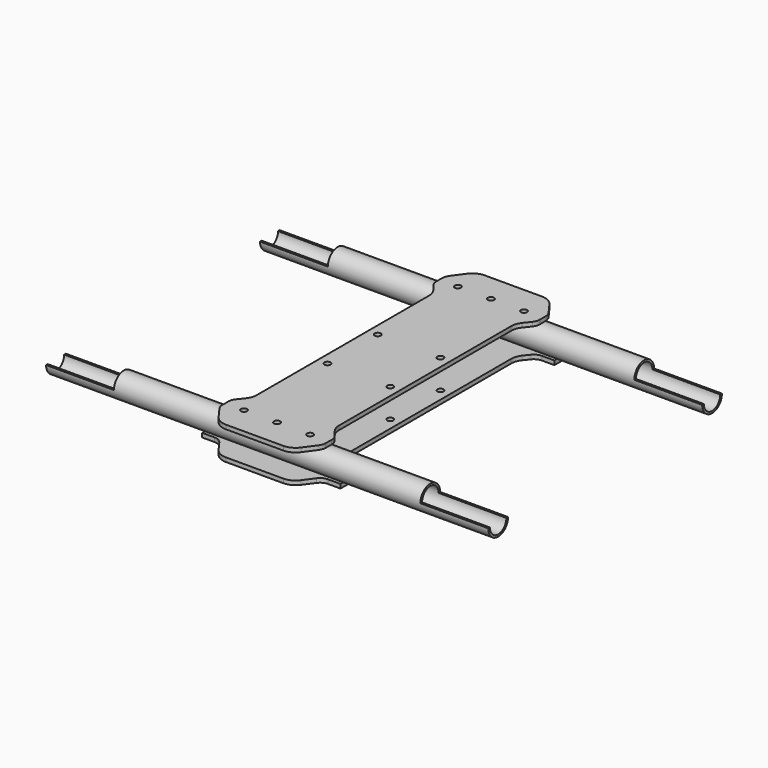
from build123d import *

# Parameters (mm, degrees)
F1_R     = 6
F1_R_2   = 5
F2_DEPTH = 107.5
F4_START = -6
F3_R     = 1.5
F4_DEPTH = 2
F6_START = 6
F5_R     = 1.5
F6_DEPTH = 2
F7_W     = 33
F7_H     = 12
F8_DEPTH = 6
F9_R     = 5
F9_2_R   = 5
F10_R    = 7.4575999994
F10_2_R  = 7.4575999994


with BuildPart() as f2:
    # F1 (on Right) → F2 (new body, symmetric)
    with BuildSketch(Plane.YZ):
        with Locations((-65, 0)):
            Circle(F1_R)
        with Locations((-65, 0)):
            Circle(F1_R_2, mode=Mode.SUBTRACT)
    extrude(amount=F2_DEPTH, both=True)


with BuildPart() as f2b:
    # F1 (on Right) → F2, piece 2 (new body, symmetric)
    with BuildSketch(Plane.YZ):
        with Locations((65, 0)):
            Circle(F1_R)
        with Locations((65, 0)):
            Circle(F1_R_2, mode=Mode.SUBTRACT)
    extrude(amount=F2_DEPTH, both=True)


with BuildPart() as f4:
    # F3 (on Top) → F4 (new body)
    with BuildSketch(Plane.XY.offset(F4_START)):
        Polygon((-20, 0), (-20, -54.9247604212), (-25.1882806771, -61.5001681654), (-33.6882806771, -61.5001681654), (-33.6196620251, -68.4998318346), (-25.1196620251, -68.4998318346), (-17.7541729063, -78.6235332489), (0, -78.6235332489), (17.7541729063, -78.6235332489), (25.1196620251, -68.4998318346), (33.6196620251, -68.4998318346), (33.6882806771, -61.5001681654), (25.1882806771, -61.5001681654), (20, -54.9247604212), (20, 0), (20, 54.9247604212), (25.1882806771, 61.5001681654), (33.6882806771, 61.5001681654), (33.6196620251, 68.4998318346), (25.1196620251, 68.4998318346), (17.7541729063, 78.6235332489), (0, 78.6235332489), (-17.7541729063, 78.6235332489), (-25.1196620251, 68.4998318346), (-33.6196620251, 68.4998318346), (-33.6882806771, 61.5001681654), (-25.1882806771, 61.5001681654), (-20, 54.9247604212), align=None)
        with Locations((-16.0910124415, -65)):
            Circle(F3_R, mode=Mode.SUBTRACT)
        with Locations((-15.25, -15.25)):
            Circle(F3_R, mode=Mode.SUBTRACT)
        with Locations((0, -65)):
            Circle(F3_R, mode=Mode.SUBTRACT)
        with Locations((16.0910124415, -65)):
            Circle(F3_R, mode=Mode.SUBTRACT)
        with Locations((15.25, -15.25)):
            Circle(F3_R, mode=Mode.SUBTRACT)
        with Locations((-15.25, 15.25)):
            Circle(F3_R, mode=Mode.SUBTRACT)
        with Locations((-16.0910124415, 65)):
            Circle(F3_R, mode=Mode.SUBTRACT)
        with Locations((15.25, 15.25)):
            Circle(F3_R, mode=Mode.SUBTRACT)
        with Locations((0, 65)):
            Circle(F3_R, mode=Mode.SUBTRACT)
        with Locations((16.0910124415, 65)):
            Circle(F3_R, mode=Mode.SUBTRACT)
    extrude(amount=-F4_DEPTH)

    # F9
    f9_edges = [f4.edges().sort_by_distance(p)[0] for p in [
        (-25.119662, -68.499832, -7),
        (25.119662, -68.499832, -7),
        (25.188281, -61.500168, -7),
        (-25.188281, -61.500168, -7),
        (-25.119662, 68.499832, -7),
        (25.119662, 68.499832, -7),
        (25.188281, 61.500168, -7),
        (-25.188281, 61.500168, -7),
    ]]
    fillet(f9_edges, radius=F9_R)

    # F10
    f10_edges = [f4.edges().sort_by_distance(p)[0] for p in [
        (17.754173, 78.623533, -7),
        (-17.754173, 78.623533, -7),
        (-20, 54.92476, -7),
        (20, 54.92476, -7),
        (20, -54.92476, -7),
        (17.754173, -78.623533, -7),
        (-17.754173, -78.623533, -7),
        (-20, -54.92476, -7),
    ]]
    fillet(f10_edges, radius=F10_R)


with BuildPart() as f6:
    # F5 (on Top) → F6 (new body)
    with BuildSketch(Plane.XY.offset(F6_START)):
        Polygon((-20, 0), (-20, -54.9247604212), (-25.1882806771, -61.5001681654), (-25.1196620251, -68.4998318346), (-17.7541729063, -78.6235332489), (0, -78.6235332489), (17.7541729063, -78.6235332489), (25.1196620251, -68.4998318346), (25.1882806771, -61.5001681654), (20, -54.9247604212), (20, 0), (20, 54.9247604212), (25.1882806771, 61.5001681654), (25.1196620251, 68.4998318346), (17.7541729063, 78.6235332489), (0, 78.6235332489), (-17.7541729063, 78.6235332489), (-25.1196620251, 68.4998318346), (-25.1882806771, 61.5001681654), (-20, 54.9247604212), align=None)
        with Locations((-16.0910124415, -65)):
            Circle(F5_R, mode=Mode.SUBTRACT)
        with Locations((-15.25, -15.25)):
            Circle(F5_R, mode=Mode.SUBTRACT)
        with Locations((0, -65)):
            Circle(F5_R, mode=Mode.SUBTRACT)
        with Locations((16.0910124415, -65)):
            Circle(F5_R, mode=Mode.SUBTRACT)
        with Locations((15.25, -15.25)):
            Circle(F5_R, mode=Mode.SUBTRACT)
        with Locations((-15.25, 15.25)):
            Circle(F5_R, mode=Mode.SUBTRACT)
        with Locations((-16.0910124415, 65)):
            Circle(F5_R, mode=Mode.SUBTRACT)
        with Locations((15.25, 15.25)):
            Circle(F5_R, mode=Mode.SUBTRACT)
        with Locations((0, 65)):
            Circle(F5_R, mode=Mode.SUBTRACT)
        with Locations((16.0910124415, 65)):
            Circle(F5_R, mode=Mode.SUBTRACT)
    extrude(amount=F6_DEPTH)

    # F9#2
    f9_2_edges = [f6.edges().sort_by_distance(p)[0] for p in [
        (-25.119662, 68.499832, 7),
        (-25.188281, 61.500168, 7),
        (25.119662, 68.499832, 7),
        (25.188281, 61.500168, 7),
        (25.119662, -68.499832, 7),
        (25.188281, -61.500168, 7),
        (-25.188281, -61.500168, 7),
        (-25.119662, -68.499832, 7),
    ]]
    fillet(f9_2_edges, radius=F9_2_R)

    # F10#2
    f10_2_edges = [f6.edges().sort_by_distance(p)[0] for p in [
        (-17.754173, 78.623533, 7),
        (17.754173, 78.623533, 7),
        (20, -54.92476, 7),
        (20, 54.92476, 7),
        (17.754173, -78.623533, 7),
        (-17.754173, -78.623533, 7),
        (-20, -54.92476, 7),
        (-20, 54.92476, 7),
    ]]
    fillet(f10_2_edges, radius=F10_2_R)


with BuildPart() as f8_tool:
    # F7 (on Top) → F8 (new body)
    with BuildSketch(Plane.XY):
        with Locations((91, -65)):
            Rectangle(F7_W, F7_H)
        with Locations((-91, -65)):
            Rectangle(F7_W, F7_H)
        with Locations((91, 65)):
            Rectangle(F7_W, F7_H)
        with Locations((-91, 65)):
            Rectangle(F7_W, F7_H)
    extrude(amount=F8_DEPTH)


with BuildPart() as f2_1:
    add(f2.part)

    # F8: cut by f8_tool
    add(f8_tool.part, mode=Mode.SUBTRACT)


with BuildPart() as f2b_1:
    add(f2b.part)

    # F8: cut by f8_tool
    add(f8_tool.part, mode=Mode.SUBTRACT)


solid = Compound([f4.part, f6.part, f2_1.part, f2b_1.part])
